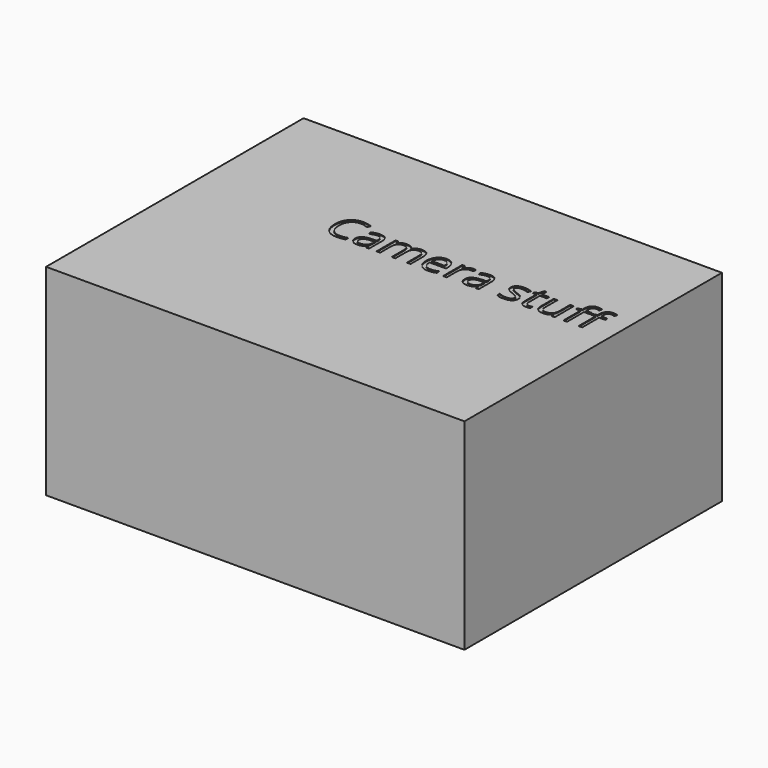
from build123d import *

# Parameters (mm, degrees)
F0_W         = 520
F0_H         = 400
F1_DEPTH     = 250
F2_TEXT_SIZE = 55.5555555556
F3_DEPTH     = 1


# Not quite as in the source:
# - Text() gives the source's letters only with a copy of the font that has no kerning and outlines rounded to 1/6400 em; it was checked with that copy


with BuildPart() as f1:
    # F0 (on Top) → F1 (new body)
    with BuildSketch(Plane.XY):
        Rectangle(F0_W, F0_H)
    extrude(amount=F1_DEPTH)

    # F2 (on face) → F3 (cut)
    with BuildSketch(Plane.XY.offset(250)):
        with Locations((-100.5757124619, 25.5601640399)):
            Text('Camera stuff', F2_TEXT_SIZE, font='Open Sans', text_align=(TextAlign.LEFT, TextAlign.BOTTOM))
    extrude(amount=-F3_DEPTH, mode=Mode.SUBTRACT)


solid = f1.part
